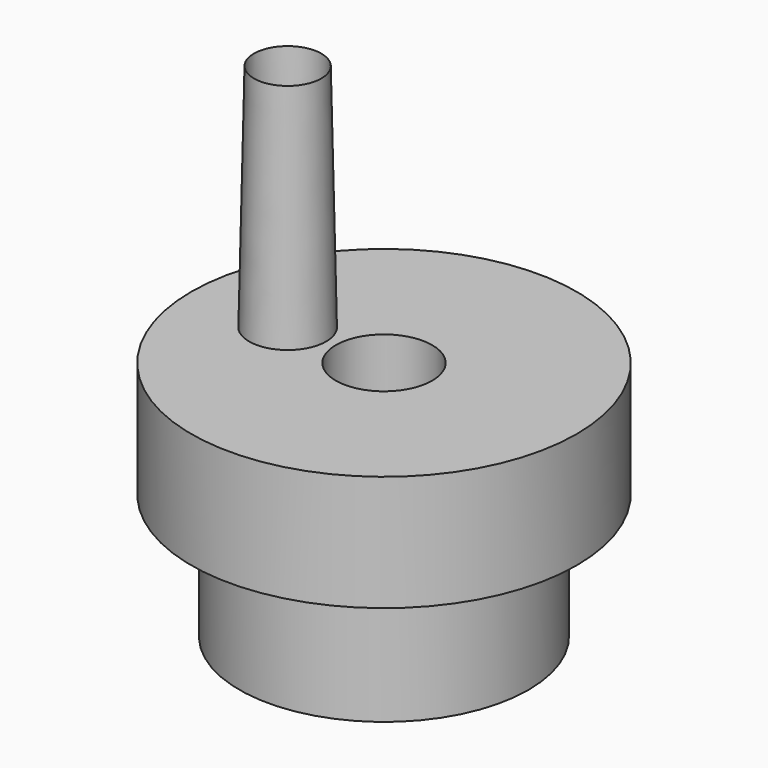
from build123d import *

# Parameters (mm, degrees)
F2_R     = 5
F3_DEPTH = 25.001
F4_R     = 3
F5_DEPTH = 25.001
F6_R     = 4
F6_R_2   = 3
F7_DEPTH = 25
F7_TAPER = 1.2


with BuildPart() as f1:
    # F0 (on Front) → F1 (revolve)
    with BuildSketch(Plane.XZ):
        Polygon((20, 0), (0, 0), (0, -25), (15, -25), (15, -1), (17.1, -1), (17.1, -12), (20, -12), align=None)
    revolve(axis=Axis((0, 0, -20.7611778751), (0, 0, -1)))

    # F2 (on Top) → F3 (cut, through all)
    with BuildSketch(Plane.XY):
        Circle(F2_R)
    extrude(amount=-F3_DEPTH, mode=Mode.SUBTRACT)

    # F4 (on face) → F5 (cut, through all)
    with BuildSketch(Plane.XY):
        with Locations((-10, 0)):
            Circle(F4_R)
    extrude(amount=-F5_DEPTH, mode=Mode.SUBTRACT)

    # F6 (on face) → F7 (join)
    with BuildSketch(Plane.XY):
        with Locations((-10, 0)):
            Circle(F6_R)
        with Locations((-10, 0)):
            Circle(F6_R_2, mode=Mode.SUBTRACT)
    extrude(amount=F7_DEPTH, taper=F7_TAPER)


solid = f1.part
